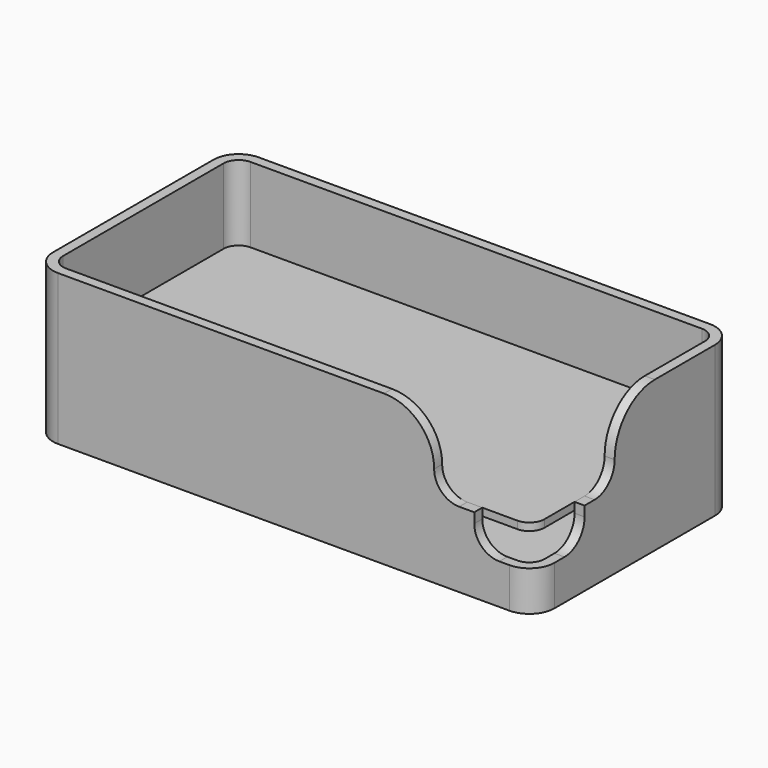
from build123d import *

# Parameters (mm, degrees)
F0_W      = 100
F0_H      = 50
F1_DEPTH  = 30
F2_R      = 5
F3_T      = -2
F4_W      = 15
F4_H      = 15
F5_DEPTH  = 20
F6_W      = 7
F6_H      = 7
F7_DEPTH  = 12.5
F11_DEPTH = 1.5
F13_R     = 10
F14_R     = 4.99999
F15_R     = 5


# Not quite as in the source:
# - a fillet or chamfer is up to 0.001 mm smaller than in the source, because OpenCascade refuses the exact size
# - a feature of the source that left no trace in its solid (it failed there, or was rolled back) is left out


with BuildPart() as f1:
    # F0 (on Top) → F1 (new body)
    with BuildSketch(Plane.XY):
        Rectangle(F0_W, F0_H)
    extrude(amount=F1_DEPTH)

    # F2
    f2_edges = [f1.edges().sort_by_distance(p)[0] for p in [
        (50, -25, 15),
        (50, 25, 15),
        (-50, -25, 15),
        (-50, 25, 15),
    ]]
    fillet(f2_edges, radius=F2_R)

    # F3
    f3_openings = [f1.faces().sort_by_distance(p)[0] for p in [
        (0, 0, 30),
    ]]
    offset(amount=F3_T, openings=f3_openings)

    # F4 (on face) → F5 (cut)
    with BuildSketch(Plane.XZ.offset(25)):
        with Locations((37.5, 22.5)):
            Rectangle(F4_W, F4_H)
        Polygon((45, 30), (45, 15), (56.0200872774, 15), (56.0200872774, 39.6855616785), (30, 39.6855616785), (30, 30), align=None)
    extrude(amount=-F5_DEPTH, mode=Mode.SUBTRACT)

    # F6 (on face) → F7 (cut)
    with BuildSketch(Plane.XZ.offset(25)):
        with Locations((41.5, 11.5)):
            Rectangle(F6_W, F6_H)
        Polygon((56.9183766905, 18.8221567892), (38, 18.8221567892), (38, 15), (45, 15), (45, 8), (56.9183766905, 8), align=None)
    extrude(amount=-F7_DEPTH, mode=Mode.SUBTRACT)

    # F13
    f13_edges = [f1.edges().sort_by_distance(p)[0] for p in [
        (30, -24, 30),
        (49, -5, 30),
    ]]
    fillet(f13_edges, radius=F13_R)

    # F14 (radius 5 in the source; OpenCascade refuses exactly that, so slightly less here)
    f14_edges = [f1.edges().sort_by_distance(p)[0] for p in [
        (30, -24, 15),
        (49, -5, 15),
    ]]
    fillet(f14_edges, radius=F14_R)

    # F15
    f15_edges = [f1.edges().sort_by_distance(p)[0] for p in [
        (38, -24, 8),
        (49, -12.5, 8),
    ]]
    fillet(f15_edges, radius=F15_R)


with BuildPart() as f11:
    # F10 (on offset) → F11 (new body)
    with BuildSketch(Plane.XY.offset(15)):
        with BuildLine():
            ThreePointArc((-45, 23), (-47.1213203436, 22.1213203436), (-48, 20))
            Line((-48, 20), (-48, -20))
            ThreePointArc((-48, -20), (-47.1213203436, -22.1213203436), (-45, -23))
            Line((-45, -23), (45, -23))
            ThreePointArc((45, -23), (47.1213203436, -22.1213203436), (48, -20))
            Line((48, -20), (48, 20))
            ThreePointArc((48, 20), (47.1213203436, 22.1213203436), (45, 23))
            Line((45, 23), (-45, 23))
        make_face()
    extrude(amount=-F11_DEPTH)


solid = Compound([f1.part, f11.part])
